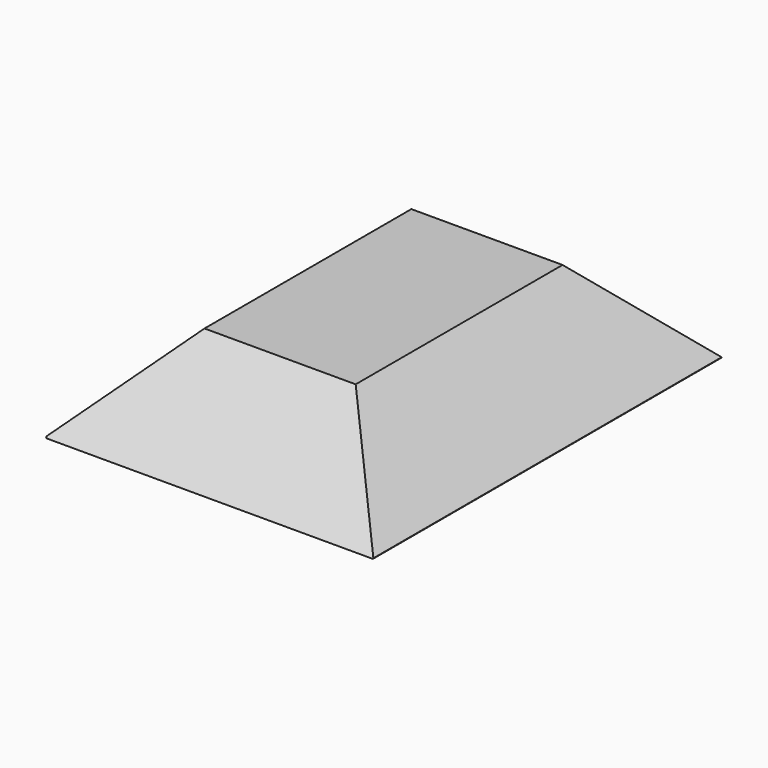
from build123d import *

# Parameters (mm, degrees)
F0_W      = 16.1028504372
F0_H      = 24.0115216002
F2_W      = 24
F2_H      = 31
F5_W      = 14.02631565
F5_H      = 35.0832007825
F6_DEPTH  = 5
F8_W      = 36.7084983736
F8_H      = 15.6723505352
F9_DEPTH  = 5
F11_W     = 29.3105235323
F11_H     = 18.8404771034
F12_DEPTH = 5
F14_W     = 31.5226018429
F14_H     = 13.2806529291
F15_DEPTH = 5
F16_W     = 23.4492318705
F16_H     = 12.546513346
F17_DEPTH = 25.4
F18_T     = 1


# Not quite as in the source:
# - a shell that OpenCascade refuses in one call is made with other operations: the cavity is built on its own and cut out


with BuildPart() as f3:
    # F0 (on Top) → F3 section 0
    with BuildSketch(Plane.XY):
        with Locations((0.0935448334, 0.0057467259)):
            Rectangle(F0_W, F0_H)
    # F2 (on offset) → F3 section 1
    with BuildSketch(Plane.XY.offset(17)):
        Rectangle(F2_W, F2_H)
    loft()

    # F5 (on face) → F6 (cut)
    with BuildSketch(Plane(origin=(-14.5, 0, 14.5), x_dir=(0.7071067812, 0, 0.7071067812), z_dir=(0.7071067812, 0, -0.7071067812))):
        with Locations((2.1269769641, -0.2655759454)):
            Rectangle(F5_W, F5_H)
    extrude(amount=F6_DEPTH, mode=Mode.SUBTRACT)

    # F8 (on face) → F9 (cut)
    with BuildSketch(Plane(origin=(14.5, 0, 14.5), x_dir=(0, 1, 0), z_dir=(0.7071067812, 0, 0.7071067812))):
        with Locations((-0.0566011295, 4.1208126349)):
            Rectangle(F8_W, F8_H)
    extrude(amount=-F9_DEPTH, mode=Mode.SUBTRACT)

    # F11 (on face) → F12 (cut)
    with BuildSketch(Plane(origin=(0, 16.25, 16.25), x_dir=(-1, 0, 0), z_dir=(0, 0.7071067812, 0.7071067812))):
        with Locations((0.3414950334, 3.7744397996)):
            Rectangle(F11_W, F11_H)
    extrude(amount=-F12_DEPTH, mode=Mode.SUBTRACT)

    # F14 (on face) → F15 (cut)
    with BuildSketch(Plane(origin=(0, -16.25, 16.25), x_dir=(1, 0, 0), z_dir=(0, 0.7071067812, -0.7071067812))):
        with Locations((0.8808970451, -0.6048630457)):
            Rectangle(F14_W, F14_H)
    extrude(amount=F15_DEPTH, mode=Mode.SUBTRACT)

    # F16 (on Front) → F17 (cut, symmetric)
    with BuildSketch(Plane.XZ):
        with Locations((-0.0993120484, 4.9331299379)):
            Rectangle(F16_W, F16_H)
    extrude(amount=F17_DEPTH, both=True, mode=Mode.SUBTRACT)

    # F18: shell of thickness 1, made by hand


with BuildPart() as f18_core1:
    # F18_t2: copy of F3
    add(f3.part)

    # the walls: a layer under each face that stays
    f18_faces = [f18_core1.faces().sort_by_distance(p)[0] for p in [
        (10.6895617231, -5.424e-06, 11.2211990551),
        (0.0256243836, -11.3257388827, 14.1031933054),
        (7.8109264385, 0, 14.1180057497),
        (0.0256243836, 11.3257388827, 14.1031933054),
        (0, 0, 17),
        (-7.7853020549, 0, 14.1436301332),
        (-10.6320571867, -1.4807e-05, 11.2468234387),
    ]]
    thicken(f18_faces, amount=-F18_T, mode=Mode.SUBTRACT)


with BuildPart() as f3_1:
    add(f3.part)

    # what is left inside the walls is the cavity
    f18_cavity = [f18_core1.part.solids().sort_by_distance(p)[0] for p in [
        (0, 4.269444, 11.216387),
    ]]
    add(f18_cavity, mode=Mode.SUBTRACT)


solid = f3_1.part
